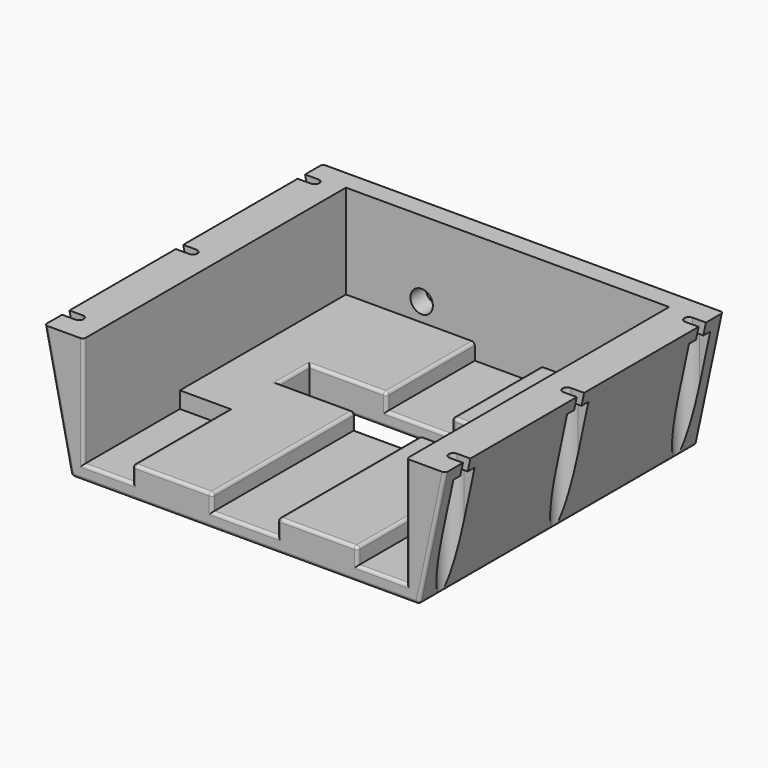
from build123d import *

# Parameters (mm, degrees)
F0_W           = 85
F0_H           = 170
F1_DEPTH       = 61
F2_W           = 79
F2_H           = 160.5
F3_DEPTH       = 46
F4_W           = 53.6
F4_H           = 19
F5_DEPTH       = 15
F6_W           = 16
F6_H           = 160.5
F6_W_2         = 24
F6_H_2         = 59
F7_DEPTH       = 8
F9_DEPTH       = 170
F11_DEPTH      = 61
F13_DEPTH      = 55
F15_T1_DEPTH   = 167.5719738762
F15_T3_DEPTH   = 74.4592516879
F15_T5_DEPTH   = 107.2
F15_T7_DEPTH   = 19
F15_T9_DEPTH   = 52.5
F15_T11_DEPTH  = 84.5
F15_T13_DEPTH  = 57.5
F15_T15_DEPTH  = 36
F15_T17_DEPTH  = 32
F15_T19_DEPTH  = 6.5
F15_T21_DEPTH  = 24
F15_T23_DEPTH  = 57.75
F15_T25_DEPTH  = 64.9058514561
F15_T27_DEPTH  = 64.9058514561
F15_T29_DEPTH  = 36
F15_T31_DEPTH  = 24
F15_T33_DEPTH  = 36.1
F15_T35_DEPTH  = 36.1
F15_T37_DEPTH  = 11.4999999105
F15_T39_DEPTH  = 69.5407484016
F15_T41_DEPTH  = 11.5
F15_T46_DEPTH  = 1.53
F15_T52_DEPTH  = 1.53
F15_T58_DEPTH  = 1.53
F15_T64_DEPTH  = 1.53
F15_S69_W      = 1.53
F15_S69_H      = 1.53
F15_T70_DEPTH  = 1.53
F15_S75_W      = 1.53
F15_S75_H      = 1.53
F15_T76_DEPTH  = 1.53
F15_S81_W      = 1.53
F15_S81_H      = 1.53
F15_T82_DEPTH  = 1.53
F15_S87_W      = 1.53
F15_S87_H      = 1.53
F15_T88_DEPTH  = 1.53
F15_S93_W      = 1.53
F15_S93_H      = 1.53
F15_T94_DEPTH  = 1.53
F15_S99_W      = 1.53
F15_S99_H      = 1.53
F15_T100_DEPTH = 1.53
F15_S105_W     = 1.53
F15_S105_H     = 1.53
F15_T106_DEPTH = 1.53
F15_S111_W     = 1.53
F15_S111_H     = 1.53
F15_T112_DEPTH = 1.53
F15_T119_DEPTH = 110.95
F15_T123_DEPTH = 22.75
F15_T130_DEPTH = 110.95
F15_T134_DEPTH = 22.75
F15_T141_DEPTH = 110.95
F15_T145_DEPTH = 22.75
F15_T152_DEPTH = 22.75
F15_T156_DEPTH = 110.95
F15_T163_DEPTH = 10.25
F15_T167_DEPTH = 35.75
F15_T174_DEPTH = 35.75
F15_T178_DEPTH = 10.25
F15_T185_DEPTH = 10.25
F15_T189_DEPTH = 27.75
F15_T196_DEPTH = 27.75
F15_T200_DEPTH = 57.75
F15_T207_DEPTH = 27.75
F15_T211_DEPTH = 10.25
F15_T218_DEPTH = 57.75
F15_T222_DEPTH = 27.75
F15_T229_DEPTH = 39.85
F15_T233_DEPTH = 22.75
F15_T240_DEPTH = 39.85
F15_T244_DEPTH = 22.75
F15_T251_DEPTH = 39.85
F15_T255_DEPTH = 22.75
F15_T262_DEPTH = 22.75
F15_T266_DEPTH = 39.85
F15_T273_DEPTH = 10.25
F15_T277_DEPTH = 35.75
F15_T284_DEPTH = 35.75
F15_T288_DEPTH = 10.25
F15_T295_DEPTH = 10.25
F15_T299_DEPTH = 35.75
F15_T306_DEPTH = 10.25
F15_T310_DEPTH = 35.75
F17_D          = 11
F18_TEXT_SIZE  = 8.5783985202
F19_DEPTH      = 1


# Not quite as in the source:
# - a fillet or chamfer that OpenCascade refuses, or shapes differently, is made with other operations: its cross-section is extruded or revolved along the edge and cut away or added
# - Text() gives the source's letters only with a copy of the font that has no kerning and outlines rounded to 1/6400 em; it was checked with that copy


with BuildPart() as f1:
    # F0 (on Top) → F1 (new body)
    with BuildSketch(Plane.XY):
        with Locations((-42.5, 2.4592517614)):
            Rectangle(F0_W, F0_H)
    extrude(amount=-F1_DEPTH)

    # F2 (on face) → F3 (cut)
    with BuildSketch(Plane.XY):
        with Locations((-39.5, -2.2907482386)):
            Rectangle(F2_W, F2_H)
    extrude(amount=-F3_DEPTH, mode=Mode.SUBTRACT)

    # F4 (on face) → F5 (cut, through all)
    with BuildSketch(Plane(origin=(0, 0, -61), x_dir=(1, 0, 0), z_dir=(0, 0, -1))):
        with Locations((-26.8, -14.4592517614)):
            Rectangle(F4_W, F4_H)
    extrude(amount=-F5_DEPTH, mode=Mode.SUBTRACT)

    # F6 (on face) → F7 (cut)
    with BuildSketch(Plane.XY.offset(-46)):
        with Locations((-8, -2.2907482386)):
            Rectangle(F6_W, F6_H)
        with Locations((-67, -53.0407482386)):
            Rectangle(F6_W_2, F6_H_2)
    extrude(amount=-F7_DEPTH, mode=Mode.SUBTRACT)

    # F8 (on face) → F9 (join, through all)
    with BuildSketch(Plane.XZ.offset(82.5407482386)):
        Polygon((-85, -61), (-85, 0), (-98, 0), align=None)
    extrude(amount=-F9_DEPTH)

    # F10 (on face) → F11 (cut, through all)
    with BuildSketch(Plane(origin=(0, 0, -61), x_dir=(1, 0, 0), z_dir=(0, 0, -1))):
        with BuildLine():
            Line((-98, -76.7092517614), (-91.5, -76.7092517614))
            ThreePointArc((-91.5, -76.7092517614), (-89.25, -74.4592517614), (-91.5, -72.2092517614))
            Line((-91.5, -72.2092517614), (-98, -72.2092517614))
            Line((-98, -72.2092517614), (-98, -76.7092517614))
        make_face()
        with BuildLine():
            Line((-98, -2.25), (-91.5, -2.25))
            ThreePointArc((-91.5, -2.25), (-89.25, 0), (-91.5, 2.25))
            Line((-91.5, 2.25), (-98, 2.25))
            Line((-98, 2.25), (-98, -2.25))
        make_face()
        with BuildLine():
            Line((-98, 67.2907482386), (-91.5, 67.2907482386))
            ThreePointArc((-91.5, 67.2907482386), (-89.25, 69.5407482386), (-91.5, 71.7907482386))
            Line((-91.5, 71.7907482386), (-98, 71.7907482386))
            Line((-98, 71.7907482386), (-98, 67.2907482386))
        make_face()
    extrude(amount=-F11_DEPTH, mode=Mode.SUBTRACT)

    # F12 (on face) → F13 (cut)
    with BuildSketch(Plane(origin=(0, 0, -61), x_dir=(1, 0, 0), z_dir=(0, 0, -1))):
        with BuildLine():
            Line((-98, -6.5), (-91.5, -6.5))
            ThreePointArc((-91.5, -6.5), (-85, 0), (-91.5, 6.5))
            Line((-91.5, 6.5), (-98, 6.5))
            Line((-98, 6.5), (-98, -6.5))
        make_face()
        with BuildLine():
            Line((-98, -80.9592517614), (-91.5, -80.9592517614))
            ThreePointArc((-91.5, -80.9592517614), (-85, -74.4592517614), (-91.5, -67.9592517614))
            Line((-91.5, -67.9592517614), (-98, -67.9592517614))
            Line((-98, -67.9592517614), (-98, -80.9592517614))
        make_face()
        with BuildLine():
            Line((-98, 63.0407482386), (-91.5, 63.0407482386))
            ThreePointArc((-91.5, 63.0407482386), (-85, 69.5407482386), (-91.5, 76.0407482386))
            Line((-91.5, 76.0407482386), (-98, 76.0407482386))
            Line((-98, 76.0407482386), (-98, 63.0407482386))
        make_face()
    extrude(amount=-F13_DEPTH, mode=Mode.SUBTRACT)

    # F14: F1 across plane


with BuildPart() as f1_1:
    add(f1.part)
    add(f1.part.mirror(Plane.YZ))

    # F15: fillet of radius 1.5 on 47 edges, made by hand

    # F15_s2 → F15_t1 (cut)
    with BuildSketch(Plane.YZ.offset(-83.7859869381)):
        with BuildLine():
            ThreePointArc((87.4592517614, -59.5), (87.0199119332, -60.5606601718), (85.9592517614, -61))
            Line((85.9592517614, -61), (87.4592517614, -61))
            Line((87.4592517614, -61), (87.4592517614, -59.5))
        make_face()
        with BuildLine():
            ThreePointArc((-82.5407482386, -59.5), (-82.1014084103, -60.5606601718), (-81.0407482386, -61))
            Line((-81.0407482386, -61), (-82.5407482386, -61))
            Line((-82.5407482386, -61), (-82.5407482386, -59.5))
        make_face()
    extrude(amount=F15_T1_DEPTH, mode=Mode.SUBTRACT)

    # F15_s4 → F15_t3 (cut)
    with BuildSketch(Plane.XZ.offset(-74.4592517614)):
        with BuildLine():
            ThreePointArc((-85.2530415919, -59.8126509918), (-84.7296562425, -60.6659709447), (-83.7859869381, -61))
            Line((-83.7859869381, -61), (-85, -61))
            Line((-85, -61), (-85.2530415919, -59.8126509918))
        make_face()
        with BuildLine():
            ThreePointArc((85.2530415919, -59.8126509918), (84.7296562425, -60.6659709447), (83.7859869381, -61))
            Line((83.7859869381, -61), (85, -61))
            Line((85, -61), (85.2530415919, -59.8126509918))
        make_face()
    extrude(amount=F15_T3_DEPTH, mode=Mode.SUBTRACT)

    # F15_s6 → F15_t5 (cut)
    with BuildSketch(Plane.YZ.offset(-53.6)):
        with BuildLine():
            ThreePointArc((23.9592517614, -59.5), (24.3985915897, -60.5606601718), (25.4592517614, -61))
            Line((25.4592517614, -61), (23.9592517614, -61))
            Line((23.9592517614, -61), (23.9592517614, -59.5))
        make_face()
        with BuildLine():
            ThreePointArc((4.9592517614, -59.5), (4.5199119332, -60.5606601718), (3.4592517614, -61))
            Line((3.4592517614, -61), (4.9592517614, -61))
            Line((4.9592517614, -61), (4.9592517614, -59.5))
        make_face()
    extrude(amount=F15_T5_DEPTH, mode=Mode.SUBTRACT)

    # F15_s8 → F15_t7 (cut)
    with BuildSketch(Plane.XZ.offset(-23.9592517614)):
        with BuildLine():
            ThreePointArc((-53.6, -59.5), (-54.0393398282, -60.5606601718), (-55.1, -61))
            Line((-55.1, -61), (-53.6, -61))
            Line((-53.6, -61), (-53.6, -59.5))
        make_face()
        with BuildLine():
            ThreePointArc((53.6, -59.5), (54.0393398282, -60.5606601718), (55.1, -61))
            Line((55.1, -61), (53.6, -61))
            Line((53.6, -61), (53.6, -59.5))
        make_face()
        with BuildLine():
            ThreePointArc((-53.6, -47.5), (-54.0393398282, -46.4393398282), (-55.1, -46))
            Line((-55.1, -46), (-53.6, -46))
            Line((-53.6, -46), (-53.6, -47.5))
        make_face()
        with BuildLine():
            ThreePointArc((53.6, -47.5), (54.0393398282, -46.4393398282), (55.1, -46))
            Line((55.1, -46), (53.6, -46))
            Line((53.6, -46), (53.6, -47.5))
        make_face()
    extrude(amount=F15_T7_DEPTH, mode=Mode.SUBTRACT)

    # F15_s10 → F15_t9 (cut)
    with BuildSketch(Plane.XZ.offset(-77.9592517614)):
        with BuildLine():
            ThreePointArc((-16, -47.5), (-16.4393398282, -46.4393398282), (-17.5, -46))
            Line((-17.5, -46), (-16, -46))
            Line((-16, -46), (-16, -47.5))
        make_face()
        with BuildLine():
            ThreePointArc((16, -47.5), (16.4393398282, -46.4393398282), (17.5, -46))
            Line((17.5, -46), (16, -46))
            Line((16, -46), (16, -47.5))
        make_face()
    extrude(amount=F15_T9_DEPTH, mode=Mode.SUBTRACT)

    # F15_s12 → F15_t11 (cut)
    with BuildSketch(Plane.XZ.offset(-3.4592517614)):
        with BuildLine():
            ThreePointArc((-17.5, -46), (-16.4393398282, -46.4393398282), (-16, -47.5))
            Line((-16, -47.5), (-16, -46))
            Line((-16, -46), (-17.5, -46))
        make_face()
        with BuildLine():
            ThreePointArc((16, -47.5), (16.4393398282, -46.4393398282), (17.5, -46))
            Line((17.5, -46), (16, -46))
            Line((16, -46), (16, -47.5))
        make_face()
    extrude(amount=F15_T11_DEPTH, mode=Mode.SUBTRACT)

    # F15_s14 → F15_t13 (cut)
    with BuildSketch(Plane.XZ.offset(23.5407482386)):
        with BuildLine():
            ThreePointArc((-55, -47.5), (-54.5606601718, -46.4393398282), (-53.5, -46))
            Line((-53.5, -46), (-55, -46))
            Line((-55, -46), (-55, -47.5))
        make_face()
        with BuildLine():
            ThreePointArc((53.5, -46), (54.5606601718, -46.4393398282), (55, -47.5))
            Line((55, -47.5), (55, -46))
            Line((55, -46), (53.5, -46))
        make_face()
    extrude(amount=F15_T13_DEPTH, mode=Mode.SUBTRACT)

    # F15_s16 → F15_t15 (cut)
    with BuildSketch(Plane.YZ.offset(-53.5)):
        with BuildLine():
            ThreePointArc((-82.5407482386, -47.5), (-82.1014084103, -46.4393398282), (-81.0407482386, -46))
            Line((-81.0407482386, -46), (-82.5407482386, -46))
            Line((-82.5407482386, -46), (-82.5407482386, -47.5))
        make_face()
    extrude(amount=F15_T15_DEPTH, mode=Mode.SUBTRACT)

    # F15_s18 → F15_t17 (cut)
    with BuildSketch(Plane.YZ.offset(-16)):
        with BuildLine():
            ThreePointArc((-82.5407482386, -55.5), (-82.1014084103, -54.4393398282), (-81.0407482386, -54))
            Line((-81.0407482386, -54), (-82.5407482386, -54))
            Line((-82.5407482386, -54), (-82.5407482386, -55.5))
        make_face()
        with BuildLine():
            ThreePointArc((4.9592517614, -55.5), (4.5199119332, -54.4393398282), (3.4592517614, -54))
            Line((3.4592517614, -54), (4.9592517614, -54))
            Line((4.9592517614, -54), (4.9592517614, -55.5))
        make_face()
        with BuildLine():
            ThreePointArc((23.9592517614, -55.5), (24.3985915897, -54.4393398282), (25.4592517614, -54))
            Line((25.4592517614, -54), (23.9592517614, -54))
            Line((23.9592517614, -54), (23.9592517614, -55.5))
        make_face()
    extrude(amount=F15_T17_DEPTH, mode=Mode.SUBTRACT)

    # F15_s20 → F15_t19 (cut)
    with BuildSketch(Plane.XY.offset(-54)):
        with BuildLine():
            ThreePointArc((-17.5, -82.5407482386), (-16.4393398282, -82.1014084103), (-16, -81.0407482386))
            Line((-16, -81.0407482386), (-16, -82.5407482386))
            Line((-16, -82.5407482386), (-17.5, -82.5407482386))
        make_face()
        with BuildLine():
            ThreePointArc((-53.5, -82.5407482386), (-54.5606601718, -82.1014084103), (-55, -81.0407482386))
            Line((-55, -81.0407482386), (-55, -82.5407482386))
            Line((-55, -82.5407482386), (-53.5, -82.5407482386))
        make_face()
        with BuildLine():
            ThreePointArc((17.5, -82.5407482386), (16.4393398282, -82.1014084103), (16, -81.0407482386))
            Line((16, -81.0407482386), (16, -82.5407482386))
            Line((16, -82.5407482386), (17.5, -82.5407482386))
        make_face()
        with BuildLine():
            ThreePointArc((53.5, -82.5407482386), (54.5606601718, -82.1014084103), (55, -81.0407482386))
            Line((55, -81.0407482386), (55, -82.5407482386))
            Line((55, -82.5407482386), (53.5, -82.5407482386))
        make_face()
        with BuildLine():
            ThreePointArc((17.5, 4.9592517614), (16.4393398282, 4.5199119332), (16, 3.4592517614))
            Line((16, 3.4592517614), (16, 4.9592517614))
            Line((16, 4.9592517614), (17.5, 4.9592517614))
        make_face()
        with BuildLine():
            ThreePointArc((-17.5, 4.9592517614), (-16.4393398282, 4.5199119332), (-16, 3.4592517614))
            Line((-16, 3.4592517614), (-16, 4.9592517614))
            Line((-16, 4.9592517614), (-17.5, 4.9592517614))
        make_face()
        with BuildLine():
            ThreePointArc((-17.5, 23.9592517614), (-16.4393398282, 24.3985915897), (-16, 25.4592517614))
            Line((-16, 25.4592517614), (-16, 23.9592517614))
            Line((-16, 23.9592517614), (-17.5, 23.9592517614))
        make_face()
        with BuildLine():
            ThreePointArc((16, 25.4592517614), (16.4393398282, 24.3985915897), (17.5, 23.9592517614))
            Line((17.5, 23.9592517614), (16, 23.9592517614))
            Line((16, 23.9592517614), (16, 25.4592517614))
        make_face()
    extrude(amount=F15_T19_DEPTH, mode=Mode.SUBTRACT)

    # F15_s22 → F15_t21 (cut)
    with BuildSketch(Plane.YZ.offset(-79)):
        with BuildLine():
            ThreePointArc((-82.5407482386, -55.5), (-82.1014084103, -54.4393398282), (-81.0407482386, -54))
            Line((-81.0407482386, -54), (-82.5407482386, -54))
            Line((-82.5407482386, -54), (-82.5407482386, -55.5))
        make_face()
    extrude(amount=F15_T21_DEPTH, mode=Mode.SUBTRACT)

    # F15_s24 → F15_t23 (cut)
    with BuildSketch(Plane.XY.offset(-54)):
        with BuildLine():
            ThreePointArc((-80.5, -82.5407482386), (-79.4393398282, -82.1014084103), (-79, -81.0407482386))
            Line((-79, -81.0407482386), (-79, -82.5407482386))
            Line((-79, -82.5407482386), (-80.5, -82.5407482386))
        make_face()
        with BuildLine():
            ThreePointArc((80.5, -82.5407482386), (79.4393398282, -82.1014084103), (79, -81.0407482386))
            Line((79, -81.0407482386), (79, -82.5407482386))
            Line((79, -82.5407482386), (80.5, -82.5407482386))
        make_face()
    extrude(amount=F15_T23_DEPTH, mode=Mode.SUBTRACT)

    # F15_s26 → F15_t25 (cut)
    with BuildSketch(Plane(origin=(5.0392110271, 0, 23.6455286654), x_dir=(0, 1, 0), z_dir=(-0.2084339945, 0, -0.9780364359))):
        with BuildLine():
            ThreePointArc((85.9592517614, 95.8475707169), (87.0199119332, 95.4082308887), (87.4592517614, 94.3475707169))
            Line((87.4592517614, 94.3475707169), (87.4592517614, 95.8475707169))
            Line((87.4592517614, 95.8475707169), (85.9592517614, 95.8475707169))
        make_face()
        with BuildLine():
            ThreePointArc((-82.5407482386, 94.3475707169), (-82.1014084103, 95.4082308887), (-81.0407482386, 95.8475707169))
            Line((-81.0407482386, 95.8475707169), (-82.5407482386, 95.8475707169))
            Line((-82.5407482386, 95.8475707169), (-82.5407482386, 94.3475707169))
        make_face()
    extrude(amount=F15_T25_DEPTH, mode=Mode.SUBTRACT)

    # F15_s28 → F15_t27 (cut)
    with BuildSketch(Plane(origin=(-5.0392110271, 0, 23.6455286654), x_dir=(0, 1, 0), z_dir=(0.2084339945, 0, -0.9780364359))):
        with BuildLine():
            ThreePointArc((87.4592517614, -94.3475707169), (87.0199119332, -95.4082308887), (85.9592517614, -95.8475707169))
            Line((85.9592517614, -95.8475707169), (87.4592517614, -95.8475707169))
            Line((87.4592517614, -95.8475707169), (87.4592517614, -94.3475707169))
        make_face()
        with BuildLine():
            ThreePointArc((-82.5407482386, -94.3475707169), (-82.1014084103, -95.4082308887), (-81.0407482386, -95.8475707169))
            Line((-81.0407482386, -95.8475707169), (-82.5407482386, -95.8475707169))
            Line((-82.5407482386, -95.8475707169), (-82.5407482386, -94.3475707169))
        make_face()
    extrude(amount=F15_T27_DEPTH, mode=Mode.SUBTRACT)

    # F15_s30 → F15_t29 (cut)
    with BuildSketch(Plane.YZ.offset(17.5)):
        with BuildLine():
            ThreePointArc((-82.5407482386, -47.5), (-82.1014084103, -46.4393398282), (-81.0407482386, -46))
            Line((-81.0407482386, -46), (-82.5407482386, -46))
            Line((-82.5407482386, -46), (-82.5407482386, -47.5))
        make_face()
    extrude(amount=F15_T29_DEPTH, mode=Mode.SUBTRACT)

    # F15_s32 → F15_t31 (cut)
    with BuildSketch(Plane.YZ.offset(55)):
        with BuildLine():
            ThreePointArc((-82.5407482386, -55.5), (-82.1014084103, -54.4393398282), (-81.0407482386, -54))
            Line((-81.0407482386, -54), (-82.5407482386, -54))
            Line((-82.5407482386, -54), (-82.5407482386, -55.5))
        make_face()
    extrude(amount=F15_T31_DEPTH, mode=Mode.SUBTRACT)

    # F15_s34 → F15_t33 (cut)
    with BuildSketch(Plane.YZ.offset(17.5)):
        with BuildLine():
            ThreePointArc((23.9592517614, -47.5), (24.3985915897, -46.4393398282), (25.4592517614, -46))
            Line((25.4592517614, -46), (23.9592517614, -46))
            Line((23.9592517614, -46), (23.9592517614, -47.5))
        make_face()
        with BuildLine():
            ThreePointArc((4.9592517614, -47.5), (4.5199119332, -46.4393398282), (3.4592517614, -46))
            Line((3.4592517614, -46), (4.9592517614, -46))
            Line((4.9592517614, -46), (4.9592517614, -47.5))
        make_face()
    extrude(amount=F15_T33_DEPTH, mode=Mode.SUBTRACT)

    # F15_s36 → F15_t35 (cut)
    with BuildSketch(Plane.YZ.offset(-53.6)):
        with BuildLine():
            ThreePointArc((23.9592517614, -47.5), (24.3985915897, -46.4393398282), (25.4592517614, -46))
            Line((25.4592517614, -46), (23.9592517614, -46))
            Line((23.9592517614, -46), (23.9592517614, -47.5))
        make_face()
        with BuildLine():
            ThreePointArc((4.9592517614, -47.5), (4.5199119332, -46.4393398282), (3.4592517614, -46))
            Line((3.4592517614, -46), (4.9592517614, -46))
            Line((4.9592517614, -46), (4.9592517614, -47.5))
        make_face()
    extrude(amount=F15_T35_DEPTH, mode=Mode.SUBTRACT)

    # F15_s38 → F15_t37 (cut)
    with BuildSketch(Plane.XZ.offset(69.540748328)):
        with BuildLine():
            ThreePointArc((85.2530415919, -59.8126509918), (84.7296562425, -60.6659709447), (83.7859869381, -61))
            Line((83.7859869381, -61), (85, -61))
            Line((85, -61), (85.2530415919, -59.8126509918))
        make_face()
        with BuildLine():
            ThreePointArc((-83.7859869381, -61), (-84.7296562425, -60.6659709447), (-85.2530415919, -59.8126509918))
            Line((-85.2530415919, -59.8126509918), (-85, -61))
            Line((-85, -61), (-83.7859869381, -61))
        make_face()
    extrude(amount=F15_T37_DEPTH, mode=Mode.SUBTRACT)

    # F15_s40 → F15_t39 (cut)
    with BuildSketch(Plane.XZ.offset(-7.35e-08)):
        with BuildLine():
            ThreePointArc((85.2530415919, -59.8126509918), (84.7296562425, -60.6659709447), (83.7859869381, -61))
            Line((83.7859869381, -61), (85, -61))
            Line((85, -61), (85.2530415919, -59.8126509918))
        make_face()
        with BuildLine():
            ThreePointArc((-85.2530415919, -59.8126509918), (-84.7296562425, -60.6659709447), (-83.7859869381, -61))
            Line((-83.7859869381, -61), (-85, -61))
            Line((-85, -61), (-85.2530415919, -59.8126509918))
        make_face()
    extrude(amount=F15_T39_DEPTH, mode=Mode.SUBTRACT)

    # F15_s42 → F15_t41 (cut)
    with BuildSketch(Plane.XZ.offset(-85.9592517614)):
        with BuildLine():
            ThreePointArc((85.2530415919, -59.8126509918), (84.7296562425, -60.6659709447), (83.7859869381, -61))
            Line((83.7859869381, -61), (85, -61))
            Line((85, -61), (85.2530415919, -59.8126509918))
        make_face()
        with BuildLine():
            ThreePointArc((-85.2530415919, -59.8126509918), (-84.7296562425, -60.6659709447), (-83.7859869381, -61))
            Line((-83.7859869381, -61), (-85, -61))
            Line((-85, -61), (-85.2530415919, -59.8126509918))
        make_face()
    extrude(amount=F15_T41_DEPTH, mode=Mode.SUBTRACT)


with BuildPart() as f15_tool44:
    # F15_s45 → F15_t46 (new body)
    with BuildSketch(Plane.XZ.offset(-85.9592517614)):
        Polygon((-83.7859869381, -59.5), (-85.282382685, -59.8189040116), (-85.0242802612, -61.03), (-83.7859869381, -61.03), align=None)
    extrude(amount=-F15_T46_DEPTH)

    # F15_s47 → F15_t48 (revolve, cut)
    with BuildSketch(Plane(origin=(-83.7859869381, 85.9592517614, -59.5), x_dir=(0.6291128696, 0, 0.7773139631), z_dir=(-0.7773139631, 0, 0.6291128696))):
        with BuildLine():
            ThreePointArc((0, -1.5), (1.5, 0), (0, 1.5))
            Line((0, 1.5), (0, -1.5))
        make_face()
    revolve(axis=Axis((-83.7859869381, 85.9592517614, -59.5), (0, 1, 0)), mode=Mode.SUBTRACT)


with BuildPart() as f1_2:
    add(f1_1.part)

    # F15_t43: cut F15_tool44
    add(f15_tool44.part, mode=Mode.SUBTRACT)


with BuildPart() as f15_tool50:
    # F15_s51 → F15_t52 (new body)
    with BuildSketch(Plane.XZ.offset(-85.9592517614)):
        Polygon((83.7859869381, -59.5), (83.7859869381, -61.03), (85.0242802612, -61.03), (85.282382685, -59.8189040116), align=None)
    extrude(amount=-F15_T52_DEPTH)

    # F15_s53 → F15_t54 (revolve, cut)
    with BuildSketch(Plane(origin=(83.7859869381, 85.9592517614, -59.5), x_dir=(-0.6291128696, 0, 0.7773139631), z_dir=(-0.7773139631, 0, -0.6291128696))):
        with BuildLine():
            ThreePointArc((0, -1.5), (1.5, 0), (0, 1.5))
            Line((0, 1.5), (0, -1.5))
        make_face()
    revolve(axis=Axis((83.7859869381, 85.9592517614, -59.5), (0, 1, 0)), mode=Mode.SUBTRACT)


with BuildPart() as f1_3:
    add(f1_2.part)

    # F15_t49: cut F15_tool50
    add(f15_tool50.part, mode=Mode.SUBTRACT)


with BuildPart() as f15_tool56:
    # F15_s57 → F15_t58 (new body)
    with BuildSketch(Plane.XZ.offset(81.0407482386)):
        Polygon((-83.7859869381, -59.5), (-85.282382685, -59.8189040116), (-85.0242802612, -61.03), (-83.7859869381, -61.03), align=None)
    extrude(amount=F15_T58_DEPTH)

    # F15_s59 → F15_t60 (revolve, cut)
    with BuildSketch(Plane(origin=(-83.7859869381, -81.0407482386, -59.5), x_dir=(0.6291128696, 0, 0.7773139631), z_dir=(0.7773139631, 0, -0.6291128696))):
        with BuildLine():
            ThreePointArc((0, -1.5), (1.5, 0), (0, 1.5))
            Line((0, 1.5), (0, -1.5))
        make_face()
    revolve(axis=Axis((-83.7859869381, -81.0407482386, -59.5), (0, -1, 0)), mode=Mode.SUBTRACT)


with BuildPart() as f1_4:
    add(f1_3.part)

    # F15_t55: cut F15_tool56
    add(f15_tool56.part, mode=Mode.SUBTRACT)


with BuildPart() as f15_tool62:
    # F15_s63 → F15_t64 (new body)
    with BuildSketch(Plane.XZ.offset(81.0407482386)):
        Polygon((83.7859869381, -59.5), (83.7859869381, -61.03), (85.0242802612, -61.03), (85.282382685, -59.8189040116), align=None)
    extrude(amount=F15_T64_DEPTH)

    # F15_s65 → F15_t66 (revolve, cut)
    with BuildSketch(Plane(origin=(83.7859869381, -81.0407482386, -59.5), x_dir=(-0.6291128696, 0, 0.7773139631), z_dir=(0.7773139631, 0, 0.6291128696))):
        with BuildLine():
            ThreePointArc((0, -1.5), (1.5, 0), (0, 1.5))
            Line((0, 1.5), (0, -1.5))
        make_face()
    revolve(axis=Axis((83.7859869381, -81.0407482386, -59.5), (0, -1, 0)), mode=Mode.SUBTRACT)


with BuildPart() as f1_5:
    add(f1_4.part)

    # F15_t61: cut F15_tool62
    add(f15_tool62.part, mode=Mode.SUBTRACT)


with BuildPart() as f15_tool68:
    # F15_s69 → F15_t70 (new body)
    with BuildSketch(Plane.YZ.offset(-17.5)):
        with Locations((24.6942517614, -46.735)):
            Rectangle(F15_S69_W, F15_S69_H)
    extrude(amount=F15_T70_DEPTH)

    # F15_s71 → F15_t72 (revolve, cut)
    with BuildSketch(Plane(origin=(-17.5, 25.4592517614, -47.5), x_dir=(0, 0.7071067812, -0.7071067812), z_dir=(0, -0.7071067812, -0.7071067812))):
        with BuildLine():
            ThreePointArc((0, -1.5), (1.5, 0), (0, 1.5))
            Line((0, 1.5), (0, -1.5))
        make_face()
    revolve(axis=Axis((-17.5, 25.4592517614, -47.5), (1, 0, 0)), mode=Mode.SUBTRACT)


with BuildPart() as f1_6:
    add(f1_5.part)

    # F15_t67: cut F15_tool68
    add(f15_tool68.part, mode=Mode.SUBTRACT)


with BuildPart() as f15_tool74:
    # F15_s75 → F15_t76 (new body)
    with BuildSketch(Plane.XY.offset(-47.5)):
        with Locations((-16.735, 4.2242517614)):
            Rectangle(F15_S75_W, F15_S75_H)
    extrude(amount=F15_T76_DEPTH)

    # F15_s77 → F15_t78 (revolve, cut)
    with BuildSketch(Plane(origin=(-17.5, 3.4592517614, -47.5), x_dir=(-0.7071067812, -0.7071067812, 0), z_dir=(-0.7071067812, 0.7071067812, 0))):
        with BuildLine():
            ThreePointArc((0, -1.5), (1.5, 0), (0, 1.5))
            Line((0, 1.5), (0, -1.5))
        make_face()
    revolve(axis=Axis((-17.5, 3.4592517614, -47.5), (0, 0, 1)), mode=Mode.SUBTRACT)


with BuildPart() as f1_7:
    add(f1_6.part)

    # F15_t73: cut F15_tool74
    add(f15_tool74.part, mode=Mode.SUBTRACT)


with BuildPart() as f15_tool80:
    # F15_s81 → F15_t82 (new body)
    with BuildSketch(Plane.XZ.offset(81.0407482386)):
        with Locations((-16.735, -46.735)):
            Rectangle(F15_S81_W, F15_S81_H)
    extrude(amount=F15_T82_DEPTH)

    # F15_s83 → F15_t84 (revolve, cut)
    with BuildSketch(Plane(origin=(-17.5, -81.0407482386, -47.5), x_dir=(-0.7071067812, 0, -0.7071067812), z_dir=(-0.7071067812, 0, 0.7071067812))):
        with BuildLine():
            ThreePointArc((0, -1.5), (1.5, 0), (0, 1.5))
            Line((0, 1.5), (0, -1.5))
        make_face()
    revolve(axis=Axis((-17.5, -81.0407482386, -47.5), (0, -1, 0)), mode=Mode.SUBTRACT)


with BuildPart() as f1_8:
    add(f1_7.part)

    # F15_t79: cut F15_tool80
    add(f15_tool80.part, mode=Mode.SUBTRACT)


with BuildPart() as f15_tool86:
    # F15_s87 → F15_t88 (new body)
    with BuildSketch(Plane.XZ.offset(81.0407482386)):
        with Locations((-54.265, -46.735)):
            Rectangle(F15_S87_W, F15_S87_H)
    extrude(amount=F15_T88_DEPTH)

    # F15_s89 → F15_t90 (revolve, cut)
    with BuildSketch(Plane(origin=(-53.5, -81.0407482386, -47.5), x_dir=(0.7071067812, 0, -0.7071067812), z_dir=(-0.7071067812, 0, -0.7071067812))):
        with BuildLine():
            ThreePointArc((0, -1.5), (1.5, 0), (0, 1.5))
            Line((0, 1.5), (0, -1.5))
        make_face()
    revolve(axis=Axis((-53.5, -81.0407482386, -47.5), (0, -1, 0)), mode=Mode.SUBTRACT)


with BuildPart() as f1_9:
    add(f1_8.part)

    # F15_t85: cut F15_tool86
    add(f15_tool86.part, mode=Mode.SUBTRACT)


with BuildPart() as f15_tool92:
    # F15_s93 → F15_t94 (new body)
    with BuildSketch(Plane.XZ.offset(81.0407482386)):
        with Locations((54.265, -46.735)):
            Rectangle(F15_S93_W, F15_S93_H)
    extrude(amount=F15_T94_DEPTH)

    # F15_s95 → F15_t96 (revolve, cut)
    with BuildSketch(Plane(origin=(53.5, -81.0407482386, -47.5), x_dir=(-0.7071067812, 0, -0.7071067812), z_dir=(-0.7071067812, 0, 0.7071067812))):
        with BuildLine():
            ThreePointArc((0, -1.5), (1.5, 0), (0, 1.5))
            Line((0, 1.5), (0, -1.5))
        make_face()
    revolve(axis=Axis((53.5, -81.0407482386, -47.5), (0, -1, 0)), mode=Mode.SUBTRACT)


with BuildPart() as f1_10:
    add(f1_9.part)

    # F15_t91: cut F15_tool92
    add(f15_tool92.part, mode=Mode.SUBTRACT)


with BuildPart() as f15_tool98:
    # F15_s99 → F15_t100 (new body)
    with BuildSketch(Plane.XZ.offset(81.0407482386)):
        with Locations((16.735, -46.735)):
            Rectangle(F15_S99_W, F15_S99_H)
    extrude(amount=F15_T100_DEPTH)

    # F15_s101 → F15_t102 (revolve, cut)
    with BuildSketch(Plane(origin=(17.5, -81.0407482386, -47.5), x_dir=(0.7071067812, 0, -0.7071067812), z_dir=(-0.7071067812, 0, -0.7071067812))):
        with BuildLine():
            ThreePointArc((0, -1.5), (1.5, 0), (0, 1.5))
            Line((0, 1.5), (0, -1.5))
        make_face()
    revolve(axis=Axis((17.5, -81.0407482386, -47.5), (0, -1, 0)), mode=Mode.SUBTRACT)


with BuildPart() as f1_11:
    add(f1_10.part)

    # F15_t97: cut F15_tool98
    add(f15_tool98.part, mode=Mode.SUBTRACT)


with BuildPart() as f15_tool104:
    # F15_s105 → F15_t106 (new body)
    with BuildSketch(Plane.YZ.offset(17.5)):
        with Locations((4.2242517614, -46.735)):
            Rectangle(F15_S105_W, F15_S105_H)
    extrude(amount=-F15_T106_DEPTH)

    # F15_s107 → F15_t108 (revolve, cut)
    with BuildSketch(Plane(origin=(17.5, 3.4592517614, -47.5), x_dir=(0, -0.7071067812, -0.7071067812), z_dir=(0, 0.7071067812, -0.7071067812))):
        with BuildLine():
            ThreePointArc((0, -1.5), (1.5, 0), (0, 1.5))
            Line((0, 1.5), (0, -1.5))
        make_face()
    revolve(axis=Axis((17.5, 3.4592517614, -47.5), (-1, 0, 0)), mode=Mode.SUBTRACT)


with BuildPart() as f1_12:
    add(f1_11.part)

    # F15_t103: cut F15_tool104
    add(f15_tool104.part, mode=Mode.SUBTRACT)


with BuildPart() as f15_tool110:
    # F15_s111 → F15_t112 (new body)
    with BuildSketch(Plane.XY.offset(-47.5)):
        with Locations((16.735, 24.6942517614)):
            Rectangle(F15_S111_W, F15_S111_H)
    extrude(amount=F15_T112_DEPTH)

    # F15_s113 → F15_t114 (revolve, cut)
    with BuildSketch(Plane(origin=(17.5, 25.4592517614, -47.5), x_dir=(0.7071067812, 0.7071067812, 0), z_dir=(0.7071067812, -0.7071067812, 0))):
        with BuildLine():
            ThreePointArc((0, -1.5), (1.5, 0), (0, 1.5))
            Line((0, 1.5), (0, -1.5))
        make_face()
    revolve(axis=Axis((17.5, 25.4592517614, -47.5), (0, 0, 1)), mode=Mode.SUBTRACT)


with BuildPart() as f1_13:
    add(f1_12.part)

    # F15_t109: cut F15_tool110
    add(f15_tool110.part, mode=Mode.SUBTRACT)


with BuildPart() as f15_tool117:
    # F15_s118 → F15_t119 (new body)
    with BuildSketch(Plane.YZ.offset(57.35)):
        with BuildLine():
            ThreePointArc((23.9592517614, -59.5), (24.3985915897, -60.5606601718), (25.4592517614, -61))
            Line((25.4592517614, -61), (23.9592517614, -61))
            Line((23.9592517614, -61), (23.9592517614, -59.5))
        make_face()
    extrude(amount=-F15_T119_DEPTH)

    split(bisect_by=Plane.YZ.offset(53.6), keep=Keep.TOP)


with BuildPart() as f15_tool121:
    # F15_s122 → F15_t123 (new body)
    with BuildSketch(Plane.XZ.offset(-4.9592517614)):
        with BuildLine():
            ThreePointArc((53.6, -59.5), (54.0393398282, -60.5606601718), (55.1, -61))
            Line((55.1, -61), (53.6, -61))
            Line((53.6, -61), (53.6, -59.5))
        make_face()
    extrude(amount=-F15_T123_DEPTH)

    split(bisect_by=Plane.XZ.offset(-23.9592517614), keep=Keep.BOTTOM)


with BuildPart() as f15_tool117_1:
    add(f15_tool117.part)

    # F15_t125: intersect F15_tool121
    add(f15_tool121.part, mode=Mode.INTERSECT)


with BuildPart() as f1_14:
    add(f1_13.part)

    # F15_t115: cut F15_tool117
    add(f15_tool117_1.part, mode=Mode.SUBTRACT)


with BuildPart() as f15_tool128:
    # F15_s129 → F15_t130 (new body)
    with BuildSketch(Plane.YZ.offset(53.6)):
        with BuildLine():
            ThreePointArc((23.9592517614, -59.5), (24.3985915897, -60.5606601718), (25.4592517614, -61))
            Line((25.4592517614, -61), (23.9592517614, -61))
            Line((23.9592517614, -61), (23.9592517614, -59.5))
        make_face()
    extrude(amount=-F15_T130_DEPTH)

    split(bisect_by=Plane.YZ.offset(-53.6), keep=Keep.BOTTOM)


with BuildPart() as f15_tool132:
    # F15_s133 → F15_t134 (new body)
    with BuildSketch(Plane.XZ.offset(-4.9592517614)):
        with BuildLine():
            ThreePointArc((-53.6, -59.5), (-54.0393398282, -60.5606601718), (-55.1, -61))
            Line((-55.1, -61), (-53.6, -61))
            Line((-53.6, -61), (-53.6, -59.5))
        make_face()
    extrude(amount=-F15_T134_DEPTH)

    split(bisect_by=Plane.XZ.offset(-23.9592517614), keep=Keep.BOTTOM)


with BuildPart() as f15_tool128_1:
    add(f15_tool128.part)

    # F15_t136: intersect F15_tool132
    add(f15_tool132.part, mode=Mode.INTERSECT)


with BuildPart() as f1_15:
    add(f1_14.part)

    # F15_t126: cut F15_tool128
    add(f15_tool128_1.part, mode=Mode.SUBTRACT)


with BuildPart() as f15_tool139:
    # F15_s140 → F15_t141 (new body)
    with BuildSketch(Plane.YZ.offset(-57.35)):
        with BuildLine():
            ThreePointArc((4.9592517614, -59.5), (4.5199119332, -60.5606601718), (3.4592517614, -61))
            Line((3.4592517614, -61), (4.9592517614, -61))
            Line((4.9592517614, -61), (4.9592517614, -59.5))
        make_face()
    extrude(amount=F15_T141_DEPTH)

    split(bisect_by=Plane.YZ.offset(-53.6), keep=Keep.BOTTOM)


with BuildPart() as f15_tool143:
    # F15_s144 → F15_t145 (new body)
    with BuildSketch(Plane.XZ.offset(-1.2092517614)):
        with BuildLine():
            ThreePointArc((-53.6, -59.5), (-54.0393398282, -60.5606601718), (-55.1, -61))
            Line((-55.1, -61), (-53.6, -61))
            Line((-53.6, -61), (-53.6, -59.5))
        make_face()
    extrude(amount=-F15_T145_DEPTH)

    split(bisect_by=Plane.XZ.offset(-4.9592517614), keep=Keep.TOP)


with BuildPart() as f15_tool139_1:
    add(f15_tool139.part)

    # F15_t147: intersect F15_tool143
    add(f15_tool143.part, mode=Mode.INTERSECT)


with BuildPart() as f1_16:
    add(f1_15.part)

    # F15_t137: cut F15_tool139
    add(f15_tool139_1.part, mode=Mode.SUBTRACT)


with BuildPart() as f15_tool150:
    # F15_s151 → F15_t152 (new body)
    with BuildSketch(Plane.XZ.offset(-1.2092517614)):
        with BuildLine():
            ThreePointArc((53.6, -59.5), (54.0393398282, -60.5606601718), (55.1, -61))
            Line((55.1, -61), (53.6, -61))
            Line((53.6, -61), (53.6, -59.5))
        make_face()
    extrude(amount=-F15_T152_DEPTH)

    split(bisect_by=Plane.XZ.offset(-4.9592517614), keep=Keep.TOP)


with BuildPart() as f15_tool154:
    # F15_s155 → F15_t156 (new body)
    with BuildSketch(Plane.YZ.offset(-53.6)):
        with BuildLine():
            ThreePointArc((4.9592517614, -59.5), (4.5199119332, -60.5606601718), (3.4592517614, -61))
            Line((3.4592517614, -61), (4.9592517614, -61))
            Line((4.9592517614, -61), (4.9592517614, -59.5))
        make_face()
    extrude(amount=F15_T156_DEPTH)

    split(bisect_by=Plane.YZ.offset(53.6), keep=Keep.TOP)


with BuildPart() as f15_tool150_1:
    add(f15_tool150.part)

    # F15_t158: intersect F15_tool154
    add(f15_tool154.part, mode=Mode.INTERSECT)


with BuildPart() as f1_17:
    add(f1_16.part)

    # F15_t148: cut F15_tool150
    add(f15_tool150_1.part, mode=Mode.SUBTRACT)


with BuildPart() as f15_tool161:
    # F15_s162 → F15_t163 (new body)
    with BuildSketch(Plane.XY.offset(-47.5)):
        with BuildLine():
            ThreePointArc((17.5, -82.5407482386), (16.4393398282, -82.1014084103), (16, -81.0407482386))
            Line((16, -81.0407482386), (16, -82.5407482386))
            Line((16, -82.5407482386), (17.5, -82.5407482386))
        make_face()
    extrude(amount=-F15_T163_DEPTH)

    split(bisect_by=Plane.XY.offset(-54), keep=Keep.BOTTOM)


with BuildPart() as f15_tool165:
    # F15_s166 → F15_t167 (new body)
    with BuildSketch(Plane.YZ.offset(19.75)):
        with BuildLine():
            ThreePointArc((-82.5407482386, -55.5), (-82.1014084103, -54.4393398282), (-81.0407482386, -54))
            Line((-81.0407482386, -54), (-82.5407482386, -54))
            Line((-82.5407482386, -54), (-82.5407482386, -55.5))
        make_face()
    extrude(amount=-F15_T167_DEPTH)

    split(bisect_by=Plane.YZ.offset(16), keep=Keep.TOP)


with BuildPart() as f15_tool161_1:
    add(f15_tool161.part)

    # F15_t169: intersect F15_tool165
    add(f15_tool165.part, mode=Mode.INTERSECT)


with BuildPart() as f1_18:
    add(f1_17.part)

    # F15_t159: cut F15_tool161
    add(f15_tool161_1.part, mode=Mode.SUBTRACT)


with BuildPart() as f15_tool172:
    # F15_s173 → F15_t174 (new body)
    with BuildSketch(Plane.YZ.offset(16)):
        with BuildLine():
            ThreePointArc((-82.5407482386, -55.5), (-82.1014084103, -54.4393398282), (-81.0407482386, -54))
            Line((-81.0407482386, -54), (-82.5407482386, -54))
            Line((-82.5407482386, -54), (-82.5407482386, -55.5))
        make_face()
    extrude(amount=-F15_T174_DEPTH)

    split(bisect_by=Plane.YZ.offset(-16), keep=Keep.BOTTOM)


with BuildPart() as f15_tool176:
    # F15_s177 → F15_t178 (new body)
    with BuildSketch(Plane.XY.offset(-47.5)):
        with BuildLine():
            ThreePointArc((-17.5, -82.5407482386), (-16.4393398282, -82.1014084103), (-16, -81.0407482386))
            Line((-16, -81.0407482386), (-16, -82.5407482386))
            Line((-16, -82.5407482386), (-17.5, -82.5407482386))
        make_face()
    extrude(amount=-F15_T178_DEPTH)

    split(bisect_by=Plane.XY.offset(-54), keep=Keep.BOTTOM)


with BuildPart() as f15_tool172_1:
    add(f15_tool172.part)

    # F15_t180: intersect F15_tool176
    add(f15_tool176.part, mode=Mode.INTERSECT)


with BuildPart() as f1_19:
    add(f1_18.part)

    # F15_t170: cut F15_tool172
    add(f15_tool172_1.part, mode=Mode.SUBTRACT)


with BuildPart() as f15_tool183:
    # F15_s184 → F15_t185 (new body)
    with BuildSketch(Plane.XY.offset(-47.5)):
        with BuildLine():
            ThreePointArc((-53.5, -82.5407482386), (-54.5606601718, -82.1014084103), (-55, -81.0407482386))
            Line((-55, -81.0407482386), (-55, -82.5407482386))
            Line((-55, -82.5407482386), (-53.5, -82.5407482386))
        make_face()
    extrude(amount=-F15_T185_DEPTH)

    split(bisect_by=Plane.XY.offset(-54), keep=Keep.BOTTOM)


with BuildPart() as f15_tool187:
    # F15_s188 → F15_t189 (new body)
    with BuildSketch(Plane.YZ.offset(-79)):
        with BuildLine():
            ThreePointArc((-82.5407482386, -55.5), (-82.1014084103, -54.4393398282), (-81.0407482386, -54))
            Line((-81.0407482386, -54), (-82.5407482386, -54))
            Line((-82.5407482386, -54), (-82.5407482386, -55.5))
        make_face()
    extrude(amount=F15_T189_DEPTH)

    split(bisect_by=Plane.YZ.offset(-55), keep=Keep.TOP)


with BuildPart() as f15_tool183_1:
    add(f15_tool183.part)

    # F15_t191: intersect F15_tool187
    add(f15_tool187.part, mode=Mode.INTERSECT)


with BuildPart() as f1_20:
    add(f1_19.part)

    # F15_t181: cut F15_tool183
    add(f15_tool183_1.part, mode=Mode.SUBTRACT)


with BuildPart() as f15_tool194:
    # F15_s195 → F15_t196 (new body)
    with BuildSketch(Plane.YZ.offset(-82.75)):
        with BuildLine():
            ThreePointArc((-82.5407482386, -55.5), (-82.1014084103, -54.4393398282), (-81.0407482386, -54))
            Line((-81.0407482386, -54), (-82.5407482386, -54))
            Line((-82.5407482386, -54), (-82.5407482386, -55.5))
        make_face()
    extrude(amount=F15_T196_DEPTH)

    split(bisect_by=Plane.YZ.offset(-79), keep=Keep.BOTTOM)


with BuildPart() as f15_tool198:
    # F15_s199 → F15_t200 (new body)
    with BuildSketch(Plane.XY.offset(-57.75)):
        with BuildLine():
            ThreePointArc((-80.5, -82.5407482386), (-79.4393398282, -82.1014084103), (-79, -81.0407482386))
            Line((-79, -81.0407482386), (-79, -82.5407482386))
            Line((-79, -82.5407482386), (-80.5, -82.5407482386))
        make_face()
    extrude(amount=F15_T200_DEPTH)

    split(bisect_by=Plane.XY.offset(-54), keep=Keep.BOTTOM)


with BuildPart() as f15_tool194_1:
    add(f15_tool194.part)

    # F15_t202: intersect F15_tool198
    add(f15_tool198.part, mode=Mode.INTERSECT)


with BuildPart() as f1_21:
    add(f1_20.part)

    # F15_t192: cut F15_tool194
    add(f15_tool194_1.part, mode=Mode.SUBTRACT)


with BuildPart() as f15_tool205:
    # F15_s206 → F15_t207 (new body)
    with BuildSketch(Plane.YZ.offset(79)):
        with BuildLine():
            ThreePointArc((-82.5407482386, -55.5), (-82.1014084103, -54.4393398282), (-81.0407482386, -54))
            Line((-81.0407482386, -54), (-82.5407482386, -54))
            Line((-82.5407482386, -54), (-82.5407482386, -55.5))
        make_face()
    extrude(amount=-F15_T207_DEPTH)

    split(bisect_by=Plane.YZ.offset(55), keep=Keep.BOTTOM)


with BuildPart() as f15_tool209:
    # F15_s210 → F15_t211 (new body)
    with BuildSketch(Plane.XY.offset(-47.5)):
        with BuildLine():
            ThreePointArc((53.5, -82.5407482386), (54.5606601718, -82.1014084103), (55, -81.0407482386))
            Line((55, -81.0407482386), (55, -82.5407482386))
            Line((55, -82.5407482386), (53.5, -82.5407482386))
        make_face()
    extrude(amount=-F15_T211_DEPTH)

    split(bisect_by=Plane.XY.offset(-54), keep=Keep.BOTTOM)


with BuildPart() as f15_tool205_1:
    add(f15_tool205.part)

    # F15_t213: intersect F15_tool209
    add(f15_tool209.part, mode=Mode.INTERSECT)


with BuildPart() as f1_22:
    add(f1_21.part)

    # F15_t203: cut F15_tool205
    add(f15_tool205_1.part, mode=Mode.SUBTRACT)


with BuildPart() as f15_tool216:
    # F15_s217 → F15_t218 (new body)
    with BuildSketch(Plane.XY.offset(-57.75)):
        with BuildLine():
            ThreePointArc((80.5, -82.5407482386), (79.4393398282, -82.1014084103), (79, -81.0407482386))
            Line((79, -81.0407482386), (79, -82.5407482386))
            Line((79, -82.5407482386), (80.5, -82.5407482386))
        make_face()
    extrude(amount=F15_T218_DEPTH)

    split(bisect_by=Plane.XY.offset(-54), keep=Keep.BOTTOM)


with BuildPart() as f15_tool220:
    # F15_s221 → F15_t222 (new body)
    with BuildSketch(Plane.YZ.offset(82.75)):
        with BuildLine():
            ThreePointArc((-82.5407482386, -55.5), (-82.1014084103, -54.4393398282), (-81.0407482386, -54))
            Line((-81.0407482386, -54), (-82.5407482386, -54))
            Line((-82.5407482386, -54), (-82.5407482386, -55.5))
        make_face()
    extrude(amount=-F15_T222_DEPTH)

    split(bisect_by=Plane.YZ.offset(79), keep=Keep.TOP)


with BuildPart() as f15_tool216_1:
    add(f15_tool216.part)

    # F15_t224: intersect F15_tool220
    add(f15_tool220.part, mode=Mode.INTERSECT)


with BuildPart() as f1_23:
    add(f1_22.part)

    # F15_t214: cut F15_tool216
    add(f15_tool216_1.part, mode=Mode.SUBTRACT)


with BuildPart() as f15_tool227:
    # F15_s228 → F15_t229 (new body)
    with BuildSketch(Plane.YZ.offset(57.35)):
        with BuildLine():
            ThreePointArc((23.9592517614, -47.5), (24.3985915897, -46.4393398282), (25.4592517614, -46))
            Line((25.4592517614, -46), (23.9592517614, -46))
            Line((23.9592517614, -46), (23.9592517614, -47.5))
        make_face()
    extrude(amount=-F15_T229_DEPTH)

    split(bisect_by=Plane.YZ.offset(53.6), keep=Keep.TOP)


with BuildPart() as f15_tool231:
    # F15_s232 → F15_t233 (new body)
    with BuildSketch(Plane.XZ.offset(-4.9592517614)):
        with BuildLine():
            ThreePointArc((53.6, -47.5), (54.0393398282, -46.4393398282), (55.1, -46))
            Line((55.1, -46), (53.6, -46))
            Line((53.6, -46), (53.6, -47.5))
        make_face()
    extrude(amount=-F15_T233_DEPTH)

    split(bisect_by=Plane.XZ.offset(-23.9592517614), keep=Keep.BOTTOM)


with BuildPart() as f15_tool227_1:
    add(f15_tool227.part)

    # F15_t235: intersect F15_tool231
    add(f15_tool231.part, mode=Mode.INTERSECT)


with BuildPart() as f1_24:
    add(f1_23.part)

    # F15_t225: cut F15_tool227
    add(f15_tool227_1.part, mode=Mode.SUBTRACT)


with BuildPart() as f15_tool238:
    # F15_s239 → F15_t240 (new body)
    with BuildSketch(Plane.YZ.offset(-57.35)):
        with BuildLine():
            ThreePointArc((23.9592517614, -47.5), (24.3985915897, -46.4393398282), (25.4592517614, -46))
            Line((25.4592517614, -46), (23.9592517614, -46))
            Line((23.9592517614, -46), (23.9592517614, -47.5))
        make_face()
    extrude(amount=F15_T240_DEPTH)

    split(bisect_by=Plane.YZ.offset(-53.6), keep=Keep.BOTTOM)


with BuildPart() as f15_tool242:
    # F15_s243 → F15_t244 (new body)
    with BuildSketch(Plane.XZ.offset(-4.9592517614)):
        with BuildLine():
            ThreePointArc((-53.6, -47.5), (-54.0393398282, -46.4393398282), (-55.1, -46))
            Line((-55.1, -46), (-53.6, -46))
            Line((-53.6, -46), (-53.6, -47.5))
        make_face()
    extrude(amount=-F15_T244_DEPTH)

    split(bisect_by=Plane.XZ.offset(-23.9592517614), keep=Keep.BOTTOM)


with BuildPart() as f15_tool238_1:
    add(f15_tool238.part)

    # F15_t246: intersect F15_tool242
    add(f15_tool242.part, mode=Mode.INTERSECT)


with BuildPart() as f1_25:
    add(f1_24.part)

    # F15_t236: cut F15_tool238
    add(f15_tool238_1.part, mode=Mode.SUBTRACT)


with BuildPart() as f15_tool249:
    # F15_s250 → F15_t251 (new body)
    with BuildSketch(Plane.YZ.offset(-17.5)):
        with BuildLine():
            ThreePointArc((4.9592517614, -47.5), (4.5199119332, -46.4393398282), (3.4592517614, -46))
            Line((3.4592517614, -46), (4.9592517614, -46))
            Line((4.9592517614, -46), (4.9592517614, -47.5))
        make_face()
    extrude(amount=-F15_T251_DEPTH)

    split(bisect_by=Plane.YZ.offset(-53.6), keep=Keep.BOTTOM)


with BuildPart() as f15_tool253:
    # F15_s254 → F15_t255 (new body)
    with BuildSketch(Plane.XZ.offset(-1.2092517614)):
        with BuildLine():
            ThreePointArc((-53.6, -47.5), (-54.0393398282, -46.4393398282), (-55.1, -46))
            Line((-55.1, -46), (-53.6, -46))
            Line((-53.6, -46), (-53.6, -47.5))
        make_face()
    extrude(amount=-F15_T255_DEPTH)

    split(bisect_by=Plane.XZ.offset(-4.9592517614), keep=Keep.TOP)


with BuildPart() as f15_tool249_1:
    add(f15_tool249.part)

    # F15_t257: intersect F15_tool253
    add(f15_tool253.part, mode=Mode.INTERSECT)


with BuildPart() as f1_26:
    add(f1_25.part)

    # F15_t247: cut F15_tool249
    add(f15_tool249_1.part, mode=Mode.SUBTRACT)


with BuildPart() as f15_tool260:
    # F15_s261 → F15_t262 (new body)
    with BuildSketch(Plane.XZ.offset(-1.2092517614)):
        with BuildLine():
            ThreePointArc((53.6, -47.5), (54.0393398282, -46.4393398282), (55.1, -46))
            Line((55.1, -46), (53.6, -46))
            Line((53.6, -46), (53.6, -47.5))
        make_face()
    extrude(amount=-F15_T262_DEPTH)

    split(bisect_by=Plane.XZ.offset(-4.9592517614), keep=Keep.TOP)


with BuildPart() as f15_tool264:
    # F15_s265 → F15_t266 (new body)
    with BuildSketch(Plane.YZ.offset(17.5)):
        with BuildLine():
            ThreePointArc((4.9592517614, -47.5), (4.5199119332, -46.4393398282), (3.4592517614, -46))
            Line((3.4592517614, -46), (4.9592517614, -46))
            Line((4.9592517614, -46), (4.9592517614, -47.5))
        make_face()
    extrude(amount=F15_T266_DEPTH)

    split(bisect_by=Plane.YZ.offset(53.6), keep=Keep.TOP)


with BuildPart() as f15_tool260_1:
    add(f15_tool260.part)

    # F15_t268: intersect F15_tool264
    add(f15_tool264.part, mode=Mode.INTERSECT)


with BuildPart() as f1_27:
    add(f1_26.part)

    # F15_t258: cut F15_tool260
    add(f15_tool260_1.part, mode=Mode.SUBTRACT)


with BuildPart() as f15_tool271:
    # F15_s272 → F15_t273 (new body)
    with BuildSketch(Plane.XY.offset(-47.5)):
        with BuildLine():
            ThreePointArc((17.5, 4.9592517614), (16.4393398282, 4.5199119332), (16, 3.4592517614))
            Line((16, 3.4592517614), (16, 4.9592517614))
            Line((16, 4.9592517614), (17.5, 4.9592517614))
        make_face()
    extrude(amount=-F15_T273_DEPTH)

    split(bisect_by=Plane.XY.offset(-54), keep=Keep.BOTTOM)


with BuildPart() as f15_tool275:
    # F15_s276 → F15_t277 (new body)
    with BuildSketch(Plane.YZ.offset(19.75)):
        with BuildLine():
            ThreePointArc((4.9592517614, -55.5), (4.5199119332, -54.4393398282), (3.4592517614, -54))
            Line((3.4592517614, -54), (4.9592517614, -54))
            Line((4.9592517614, -54), (4.9592517614, -55.5))
        make_face()
    extrude(amount=-F15_T277_DEPTH)

    split(bisect_by=Plane.YZ.offset(16), keep=Keep.TOP)


with BuildPart() as f15_tool271_1:
    add(f15_tool271.part)

    # F15_t279: intersect F15_tool275
    add(f15_tool275.part, mode=Mode.INTERSECT)


with BuildPart() as f1_28:
    add(f1_27.part)

    # F15_t269: cut F15_tool271
    add(f15_tool271_1.part, mode=Mode.SUBTRACT)


with BuildPart() as f15_tool282:
    # F15_s283 → F15_t284 (new body)
    with BuildSketch(Plane.YZ.offset(16)):
        with BuildLine():
            ThreePointArc((4.9592517614, -55.5), (4.5199119332, -54.4393398282), (3.4592517614, -54))
            Line((3.4592517614, -54), (4.9592517614, -54))
            Line((4.9592517614, -54), (4.9592517614, -55.5))
        make_face()
    extrude(amount=-F15_T284_DEPTH)

    split(bisect_by=Plane.YZ.offset(-16), keep=Keep.BOTTOM)


with BuildPart() as f15_tool286:
    # F15_s287 → F15_t288 (new body)
    with BuildSketch(Plane.XY.offset(-47.5)):
        with BuildLine():
            ThreePointArc((-17.5, 4.9592517614), (-16.4393398282, 4.5199119332), (-16, 3.4592517614))
            Line((-16, 3.4592517614), (-16, 4.9592517614))
            Line((-16, 4.9592517614), (-17.5, 4.9592517614))
        make_face()
    extrude(amount=-F15_T288_DEPTH)

    split(bisect_by=Plane.XY.offset(-54), keep=Keep.BOTTOM)


with BuildPart() as f15_tool282_1:
    add(f15_tool282.part)

    # F15_t290: intersect F15_tool286
    add(f15_tool286.part, mode=Mode.INTERSECT)


with BuildPart() as f1_29:
    add(f1_28.part)

    # F15_t280: cut F15_tool282
    add(f15_tool282_1.part, mode=Mode.SUBTRACT)


with BuildPart() as f15_tool293:
    # F15_s294 → F15_t295 (new body)
    with BuildSketch(Plane.XY.offset(-57.75)):
        with BuildLine():
            ThreePointArc((-17.5, 23.9592517614), (-16.4393398282, 24.3985915897), (-16, 25.4592517614))
            Line((-16, 25.4592517614), (-16, 23.9592517614))
            Line((-16, 23.9592517614), (-17.5, 23.9592517614))
        make_face()
    extrude(amount=F15_T295_DEPTH)

    split(bisect_by=Plane.XY.offset(-54), keep=Keep.BOTTOM)


with BuildPart() as f15_tool297:
    # F15_s298 → F15_t299 (new body)
    with BuildSketch(Plane.YZ.offset(16)):
        with BuildLine():
            ThreePointArc((23.9592517614, -55.5), (24.3985915897, -54.4393398282), (25.4592517614, -54))
            Line((25.4592517614, -54), (23.9592517614, -54))
            Line((23.9592517614, -54), (23.9592517614, -55.5))
        make_face()
    extrude(amount=-F15_T299_DEPTH)

    split(bisect_by=Plane.YZ.offset(-16), keep=Keep.BOTTOM)


with BuildPart() as f15_tool293_1:
    add(f15_tool293.part)

    # F15_t301: intersect F15_tool297
    add(f15_tool297.part, mode=Mode.INTERSECT)


with BuildPart() as f1_30:
    add(f1_29.part)

    # F15_t291: cut F15_tool293
    add(f15_tool293_1.part, mode=Mode.SUBTRACT)


with BuildPart() as f15_tool304:
    # F15_s305 → F15_t306 (new body)
    with BuildSketch(Plane.XY.offset(-57.75)):
        with BuildLine():
            ThreePointArc((16, 25.4592517614), (16.4393398282, 24.3985915897), (17.5, 23.9592517614))
            Line((17.5, 23.9592517614), (16, 23.9592517614))
            Line((16, 23.9592517614), (16, 25.4592517614))
        make_face()
    extrude(amount=F15_T306_DEPTH)

    split(bisect_by=Plane.XY.offset(-54), keep=Keep.BOTTOM)


with BuildPart() as f15_tool308:
    # F15_s309 → F15_t310 (new body)
    with BuildSketch(Plane.YZ.offset(19.75)):
        with BuildLine():
            ThreePointArc((23.9592517614, -55.5), (24.3985915897, -54.4393398282), (25.4592517614, -54))
            Line((25.4592517614, -54), (23.9592517614, -54))
            Line((23.9592517614, -54), (23.9592517614, -55.5))
        make_face()
    extrude(amount=-F15_T310_DEPTH)

    split(bisect_by=Plane.YZ.offset(16), keep=Keep.TOP)


with BuildPart() as f15_tool304_1:
    add(f15_tool304.part)

    # F15_t312: intersect F15_tool308
    add(f15_tool308.part, mode=Mode.INTERSECT)


with BuildPart() as f1_31:
    add(f1_30.part)

    # F15_t302: cut F15_tool304
    add(f15_tool304_1.part, mode=Mode.SUBTRACT)

    # F17 (through all)
    with Locations(Plane(origin=(0, 87.4592517614, 0), x_dir=(-1, 0, 0), z_dir=(0, 1, 0))):
        with Locations((42, -37)):
            Hole(F17_D / 2)

    # F18 (on face) → F19 (cut)
    with BuildSketch(Plane.XY.offset(-46)):
        with Locations((23.2473881304, 48.5797758901)):
            Text('SWS #: 0493', F18_TEXT_SIZE, font='Open Sans', font_style=FontStyle.BOLD, text_align=(TextAlign.LEFT, TextAlign.BOTTOM))
    extrude(amount=-F19_DEPTH, mode=Mode.SUBTRACT)


solid = f1_31.part
